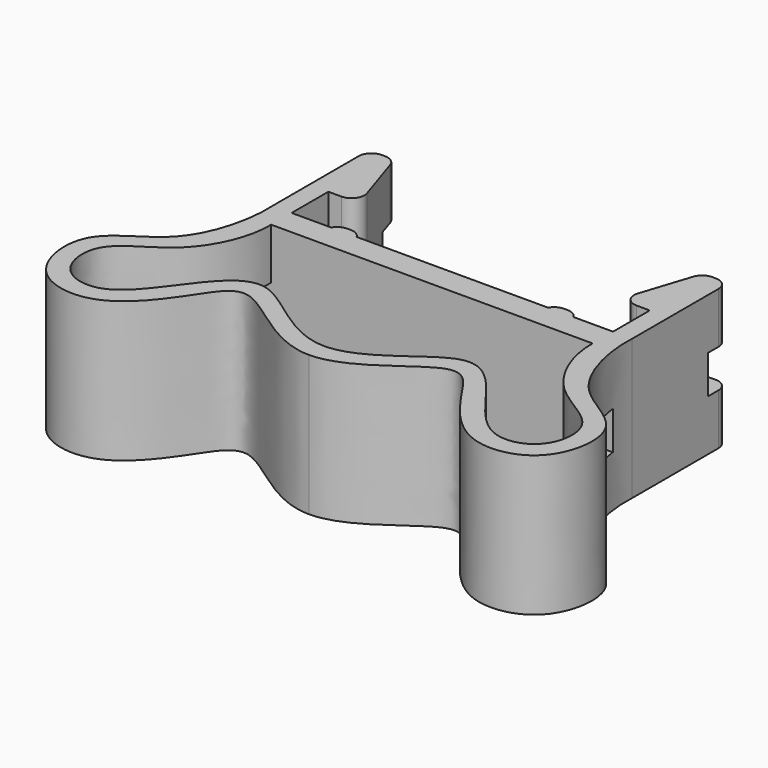
from build123d import *

# Parameters (mm, degrees)
F0_W        = 2
F0_H        = 0.5
F1_DEPTH    = 11
F2_T1_DEPTH = 17.8819096024
F2_T3_DEPTH = 16
F2_T5_DEPTH = 14.63271264
F2_T7_DEPTH = 15.3301270189
F3_W        = 2
F3_H        = 3
F4_DEPTH    = 15


# Not quite as in the source:
# - a fillet or chamfer that OpenCascade refuses, or shapes differently, is made with other operations: its cross-section is extruded or revolved along the edge and cut away or added


with BuildPart() as f1:
    # F0 (on Top) → F1 (new body)
    with BuildSketch(Plane.XY):
        with BuildLine():
            Line((-14.1, 9.4475987206), (-14.1, 0))
            add(Edge.make_bspline(
                [(-14.1, 0), (-13.9666085935, -1.9503301305), (-15.0750300263, -7.6287393484), (-21.3730788003, -9.3291396524), (-20.4128316218, -16.3144858473), (-14.259658092, -17.4352339168), (-10.6266757986, -12.5631403321), (-8.07173481, -8.20416774), (-3.298607474, -14.0162183623), (0, -14.0419555828)],
                knots=[0, 0, 0, 0, 0.1580523046, 0.2988042817, 0.4345842251, 0.5663505105, 0.7117959604, 0.8211329211, 1, 1, 1, 1], degree=3))
            add(Edge.make_bspline(
                [(14.1, 0), (13.9666085935, -1.9503301305), (15.0750300263, -7.6287393484), (21.3730788003, -9.3291396524), (20.4128316218, -16.3144858473), (14.259658092, -17.4352339168), (10.6266757986, -12.5631403321), (8.07173481, -8.20416774), (3.298607474, -14.0162183623), (0, -14.0419555828)],
                knots=[0, 0, 0, 0, 0.1580523046, 0.2988042817, 0.4345842251, 0.5663505105, 0.7117959604, 0.8211329211, 1, 1, 1, 1], degree=3))
            Line((14.1, 0), (14.1, 9.4475987206))
            Line((14.1, 9.4475987206), (12.1, 9.4475987206))
            Line((12.1, 9.4475987206), (10.2, 3.6))
            Line((10.2, 3.6), (12.6, 3.6))
            Line((12.6, 3.6), (12.6, 0))
            Line((12.6, 0), (9.5, 0))
            Line((9.5, 0), (7.5, 0))
            Line((7.5, 0), (0, 0))
            Line((0, 0), (-7.5, 0))
            Line((-7.5, 0), (-9.5, 0))
            Line((-9.5, 0), (-12.6, 0))
            Line((-12.6, 0), (-12.6, 3.6))
            Line((-12.6, 3.6), (-10.2, 3.6))
            Line((-10.2, 3.6), (-12.1, 9.4475987206))
            Line((-12.1, 9.4475987206), (-14.1, 9.4475987206))
        make_face()
        with BuildLine():
            add(Edge.make_bspline(
                [(-12.6, -2), (-12.5584885174, -4.0488143731), (-14.3514424803, -8.4231611099), (-19.6579670763, -10.1247790951), (-19.0854803087, -14.8444965683), (-14.951052578, -15.8383241392), (-11.9555900431, -11.5662850742), (-7.8077190594, -6.3441347041), (-3.2070761008, -12.5136579418), (0, -12.5419555828)],
                knots=[0, 0, 0, 0, 0.1589928689, 0.2993855539, 0.4170039917, 0.5292468706, 0.6723550613, 0.8117091941, 1, 1, 1, 1], degree=3))
            Line((-12.6, -2), (12.6, -2))
            add(Edge.make_bspline(
                [(12.6, -2), (12.5584885174, -4.0488143731), (14.3514424803, -8.4231611099), (19.6579670763, -10.1247790951), (19.0854803087, -14.8444965683), (14.951052578, -15.8383241392), (11.9555900431, -11.5662850742), (7.8077190594, -6.3441347041), (3.2070761008, -12.5136579418), (0, -12.5419555828)],
                knots=[0, 0, 0, 0, 0.1589928689, 0.2993855539, 0.4170039917, 0.5292468706, 0.6723550613, 0.8117091941, 1, 1, 1, 1], degree=3))
        make_face(mode=Mode.SUBTRACT)
        with Locations((-8.5, 0.25)):
            Rectangle(F0_W, F0_H)
        with Locations((8.5, 0.25)):
            Rectangle(F0_W, F0_H)
    extrude(amount=F1_DEPTH)

    # F2: fillet of radius 1 on 10 edges, made by hand

    # F2_s2 → F2_t1 (cut)
    with BuildSketch(Plane.XY.offset(-3.4409548012)):
        with BuildLine():
            ThreePointArc((-11.5763819205, 3.6), (-10.7673649261, 4.0122147477), (-10.6253254042, 4.9090169944))
            Line((-10.6253254042, 4.9090169944), (-10.2, 3.6))
            Line((-10.2, 3.6), (-11.5763819205, 3.6))
        make_face()
        with BuildLine():
            ThreePointArc((10.6253254042, 4.9090169944), (10.7673649261, 4.0122147477), (11.5763819205, 3.6))
            Line((11.5763819205, 3.6), (10.2, 3.6))
            Line((10.2, 3.6), (10.6253254042, 4.9090169944))
        make_face()
    extrude(amount=F2_T1_DEPTH, mode=Mode.SUBTRACT)

    # F2_s4 → F2_t3 (cut)
    with BuildSketch(Plane.XY.offset(-2.5)):
        with BuildLine():
            ThreePointArc((-14.1, 8.4475987206), (-13.8071067812, 9.1547055018), (-13.1, 9.4475987206))
            Line((-13.1, 9.4475987206), (-14.1, 9.4475987206))
            Line((-14.1, 9.4475987206), (-14.1, 8.4475987206))
        make_face()
        with BuildLine():
            ThreePointArc((14.1, 8.4475987206), (13.8071067812, 9.1547055018), (13.1, 9.4475987206))
            Line((13.1, 9.4475987206), (14.1, 9.4475987206))
            Line((14.1, 9.4475987206), (14.1, 8.4475987206))
        make_face()
    extrude(amount=F2_T3_DEPTH, mode=Mode.SUBTRACT)

    # F2_s6 → F2_t5 (cut)
    with BuildSketch(Plane.XY.offset(-1.81635632)):
        with BuildLine():
            ThreePointArc((-11.8754860117, 8.756615715), (-12.2387572757, 9.256615715), (-12.826542528, 9.4475987206))
            Line((-12.826542528, 9.4475987206), (-12.1, 9.4475987206))
            Line((-12.1, 9.4475987206), (-11.8754860117, 8.756615715))
        make_face()
        with BuildLine():
            ThreePointArc((12.826542528, 9.4475987206), (12.2387572757, 9.256615715), (11.8754860117, 8.756615715))
            Line((11.8754860117, 8.756615715), (12.1, 9.4475987206))
            Line((12.1, 9.4475987206), (12.826542528, 9.4475987206))
        make_face()
    extrude(amount=F2_T5_DEPTH, mode=Mode.SUBTRACT)

    # F2_s8 → F2_t7 (cut)
    with BuildSketch(Plane.XY.offset(-2.1650635095)):
        with BuildLine():
            ThreePointArc((-8.6339745962, 0.5), (-9.1339745962, 0.3660254038), (-9.5, 0))
            Line((-9.5, 0), (-9.5, 0.5))
            Line((-9.5, 0.5), (-8.6339745962, 0.5))
        make_face()
        with BuildLine():
            ThreePointArc((-7.5, 0), (-7.8660254038, 0.3660254038), (-8.3660254038, 0.5))
            Line((-8.3660254038, 0.5), (-7.5, 0.5))
            Line((-7.5, 0.5), (-7.5, 0))
        make_face()
        with BuildLine():
            ThreePointArc((8.3660254038, 0.5), (7.8660254038, 0.3660254038), (7.5, 0))
            Line((7.5, 0), (7.5, 0.5))
            Line((7.5, 0.5), (8.3660254038, 0.5))
        make_face()
        with BuildLine():
            ThreePointArc((9.5, 0), (9.1339745962, 0.3660254038), (8.6339745962, 0.5))
            Line((8.6339745962, 0.5), (9.5, 0.5))
            Line((9.5, 0.5), (9.5, 0))
        make_face()
    extrude(amount=F2_T7_DEPTH, mode=Mode.SUBTRACT)

    # F3 (on Right) → F4 (cut, symmetric)
    with BuildSketch(Plane.YZ):
        with Locations((-3, 5.5)):
            Rectangle(F3_W, F3_H)
        with Locations((8.4475987206, 5.5)):
            Rectangle(F3_W, F3_H)
    extrude(amount=F4_DEPTH, both=True, mode=Mode.SUBTRACT)


solid = f1.part
